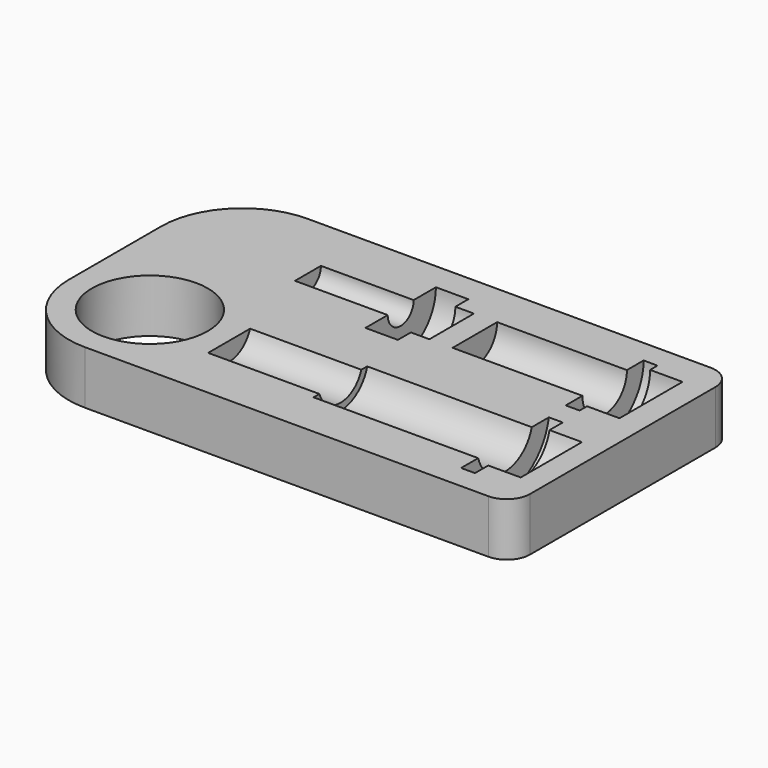
from build123d import *

# Parameters (mm, degrees)
F0_R         = 12.5
F1_DEPTH     = 11.5
F7_TEXT_SIZE = 5.5555555556
F8_DEPTH     = 1


# Not quite as in the source:
# - Text() gives the source's letters only with a copy of the font that has no kerning and outlines rounded to 1/6400 em; it was checked with that copy


with BuildPart() as f1:
    # F0 (on Top) → F1 (new body)
    with BuildSketch(Plane.XY):
        with BuildLine():
            ThreePointArc((0, 17.5), (5.1256313292, 5.1256313292), (17.5, 0))
            Line((17.5, 0), (104.5, 0))
            ThreePointArc((104.5, 0), (108.0355339059, 1.4644660941), (109.5, 5))
            Line((109.5, 5), (109.5, 55))
            ThreePointArc((109.5, 55), (108.0355339059, 58.5355339059), (104.5, 60))
            Line((104.5, 60), (17.5, 60))
            ThreePointArc((17.5, 60), (5.1256313292, 54.8743686708), (0, 42.5))
            Line((0, 42.5), (0, 17.5))
        make_face()
        with Locations((17.5, 17.5)):
            Circle(F0_R, mode=Mode.SUBTRACT)
    extrude(amount=F1_DEPTH)

    # F2 (on face) → F3 (revolve, cut)
    with BuildSketch(Plane.XY.offset(11.5)):
        Polygon((50, 44.5), (30, 44.5), (30, 41), (50, 41), (50, 35), (57, 35), (57, 38.5), (61, 38.5), (61, 44.5), (57, 44.5), align=None)
        Polygon((94, 44.5), (66, 44.5), (66, 38.5), (94, 38.5), (94, 34), (97, 34), (97, 36), (104, 36), (104, 44.5), (97, 44.5), align=None)
    revolve(axis=Axis((80, 44.5, 11.5), (1, 0, 0)), mode=Mode.SUBTRACT)

    # F5 (on offset) → F6 (revolve, cut)
    with BuildSketch(Plane.XY.offset(13.5)):
        Polygon((94.5, 17), (59, 17), (35, 17), (35, 11), (59, 11), (59, 9.5), (94.5, 9.5), (94.5, 5), (97.5, 5), (97.5, 8.5), (104.5, 8.5), (104.5, 17), (97.5, 17), align=None)
    revolve(axis=Axis((47, 17, 13.5), (1, 0, 0)), mode=Mode.SUBTRACT)

    # F7 (on face) → F8 (cut)
    with BuildSketch(Plane(origin=(0, 0, 0), x_dir=(1, 0, 0), z_dir=(0, 0, -1))):
        with Locations((30, -9)):
            Text('998, 999', F7_TEXT_SIZE, font='Open Sans', text_align=(TextAlign.LEFT, TextAlign.BOTTOM))
    extrude(amount=-F8_DEPTH, mode=Mode.SUBTRACT)


solid = f1.part
